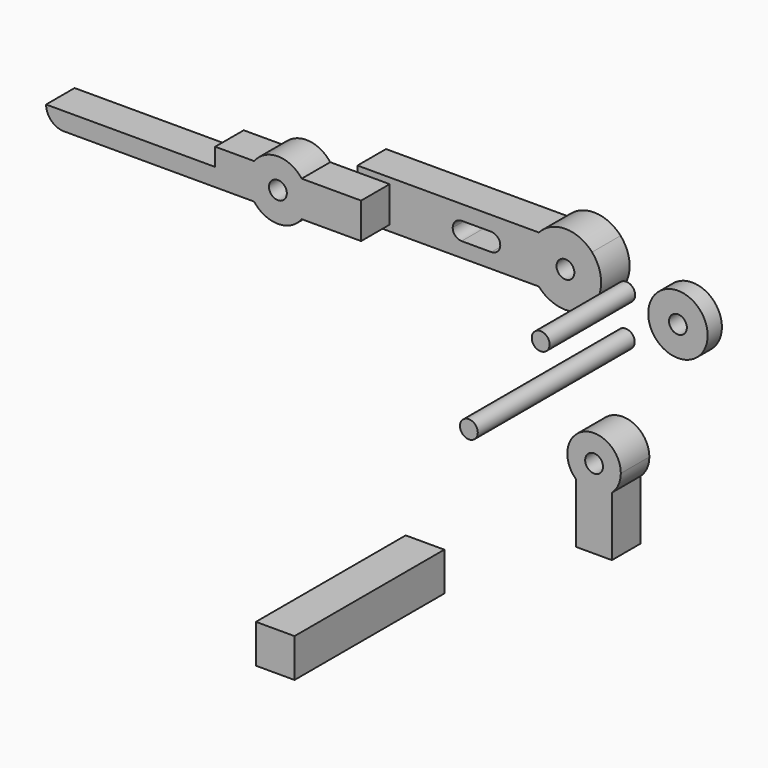
from build123d import *

# Parameters (mm, degrees)
F0_R      = 1.5
F1_DEPTH  = 6
F2_R      = 1.5
F2_W      = 5.4118521512
F2_H      = 6
F3_DEPTH  = 6
F4_R      = 5
F4_R_2    = 1.5
F5_DEPTH  = 3
F6_R      = 1.5
F7_DEPTH  = 18
F8_R      = 1.5
F9_DEPTH  = 33
F10_R     = 1.5
F10_W     = 6
F10_H     = 6
F11_DEPTH = 6
F12_DEPTH = 6
F13_W     = 6.5
F13_H     = 6.5
F14_DEPTH = 31.5


# Not quite as in the source:
# - ends of sketch curves that miss each other by under 0.0002 mm in the source are joined


with BuildPart() as f1:
    # F0 (on Front) → F1 (new body)
    with BuildSketch(Plane.XZ):
        with BuildLine():
            ThreePointArc((3.9999999804, -3.0000000261), (4.7434164851, -1.5811388455), (5, 0))
            ThreePointArc((5, 0), (4.7434164917, 1.5811388258), (4.0000000055, 2.9999999927))
            Line((3.9999999804, 2.9999999739), (3.9999999804, -3.0000000261))
        make_face()
        with BuildLine():
            ThreePointArc((4.0000000055, 2.9999999927), (4.7434164917, 1.5811388258), (5, 0))
            ThreePointArc((5, 0), (4.7434164851, -1.5811388455), (3.9999999804, -3.0000000261))
            Line((3.9999999804, -3.0000000261), (13.9999999804, -3.0000000261))
            Line((13.9999999804, -3.0000000261), (13.9999999804, 2.9999999739))
            Line((13.9999999804, 2.9999999739), (3.9999999804, 2.9999999739))
        make_face()
        with BuildLine():
            Line((3.9999999804, -3.0000000261), (3.9999999804, 2.9999999739))
            ThreePointArc((4.0000000055, 2.9999999927), (2.09e-08, 5), (-3.9999999804, 3.0000000261))
            Line((-3.9999999804, 3.0000000261), (-3.9999999804, -3.0000000261))
            ThreePointArc((-3.9999999804, -3.0000000261), (0, -5), (3.9999999804, -3.0000000261))
        make_face()
        Circle(F0_R, mode=Mode.SUBTRACT)
        with BuildLine():
            Line((-3.9999999804, -3.0000000261), (-3.9999999804, 3.0000000261))
            ThreePointArc((-3.9999999804, 3.0000000261), (-5, 0), (-3.9999999804, -3.0000000261))
        make_face()
        with BuildLine():
            ThreePointArc((-3.9999999804, -3.0000000261), (-5, 0), (-3.9999999804, 3.0000000261))
            Line((-3.9999999804, 3.0000000261), (-10.545078665, 3.0000000261))
            Line((-10.545078665, 3.0000000261), (-10.545078665, 0))
            Line((-10.545078665, 0), (-38.9999999804, 0))
            ThreePointArc((-38.9999999804, -2.61e-08), (-38.121320324, -2.1213203696), (-35.9999999804, -3.0000000261))
            Line((-35.9999999804, -3.0000000261), (-3.9999999804, -3.0000000261))
        make_face()
    extrude(amount=F1_DEPTH)

    # F2 (on face) → F3 (join)
    with BuildSketch(Plane(origin=(0, 0, 0), x_dir=(-1, 0, 0), z_dir=(0, 1, 0))):
        with BuildLine():
            ThreePointArc((-39.1041604406, 3.9999999739), (-43.5762964189, 6), (-48.0484323972, 3.9999999739))
            Line((-48.0484323972, 3.9999999739), (-39.1041604406, 3.9999999739))
        make_face()
        with BuildLine():
            Line((-39.1041606338, -4.00000019), (-48.048432204, -4.00000019))
            ThreePointArc((-48.048432204, -4.00000019), (-43.5762964189, -6), (-39.1041606338, -4.00000019))
        make_face()
        with BuildLine():
            Line((-39.1041604406, 3.9999999739), (-48.0484323972, 3.9999999739))
            ThreePointArc((-48.0484323972, 3.9999999739), (-49.5762964189, -1.449e-07), (-48.048432204, -4.00000019))
            Line((-48.048432204, -4.00000019), (-39.1041606338, -4.00000019))
            ThreePointArc((-39.1041606338, -4.00000019), (-37.9712623106, -2.1409326577), (-37.5762964189, 0))
            ThreePointArc((-37.5762964189, 0), (-37.9712622589, 2.1409325223), (-39.1041604406, 3.9999999739))
        make_face()
        with Locations((-43.5762964189, 0)):
            Circle(F2_R, mode=Mode.SUBTRACT)
        with Locations((-11.2940739049, -2.61e-08)):
            Rectangle(F2_W, F2_H)
        with BuildLine():
            Line((-8.5881474018, 3.9999999739), (-39.1041604406, 3.9999999739))
            ThreePointArc((-39.1041604406, 3.9999999739), (-37.9712622589, 2.1409325223), (-37.5762964189, 0))
            ThreePointArc((-37.5762964189, 0), (-37.9712623106, -2.1409326577), (-39.1041606338, -4.00000019))
            Line((-39.1041606338, -4.00000019), (-14.5881475508, -4.00000019))
            Line((-14.5881475508, -4.00000019), (-8.5881474018, -4.00000019))
            Line((-8.5881474018, -4.00000019), (-8.5881478293, -3.0000000261))
            Line((-8.5881478293, -3.0000000261), (-13.9999999804, -3.0000000261))
            Line((-13.9999999804, -3.0000000261), (-13.9999999804, 2.9999999739))
            Line((-13.9999999804, 2.9999999739), (-8.5881478293, 2.9999999739))
            Line((-8.5881478293, 2.9999999739), (-8.5881474018, 3.9999999739))
        make_face()
        with BuildLine():
            ThreePointArc((-24.6078900066, 1.33e-08), (-25.048135537, -1.061565088), (-26.1104506254, -1.4999978011))
            Line((-26.1104506254, -1.4999978011), (-31.1104506254, -1.4999978011))
            ThreePointArc((-31.1104506254, -1.4999978011), (-32.6104506254, 0), (-31.1104506254, 1.5))
            Line((-31.1104506254, 1.5), (-31.1104506254, 1.5137138676))
            Line((-31.1104506254, 1.5137138676), (-26.1104506254, 1.5137138676))
            Line((-26.1104506254, 1.5137138676), (-26.1104506254, 1.4999978277))
            ThreePointArc((-26.1104506254, 1.4999978277), (-25.048135537, 1.0615651145), (-24.6078900066, 1.33e-08))
        make_face(mode=Mode.SUBTRACT)
    extrude(amount=F3_DEPTH)


with BuildPart() as f5:
    # F4 (on Front) → F5 (new body)
    with BuildSketch(Plane.XZ):
        with Locations((64.899995923, 0)):
            Circle(F4_R)
        with Locations((64.899995923, 0)):
            Circle(F4_R_2, mode=Mode.SUBTRACT)
    extrude(amount=F5_DEPTH)


with BuildPart() as f7:
    # F6 (on Front) → F7 (new body)
    with BuildSketch(Plane.XZ):
        with Locations((53.8045093417, 0)):
            Circle(F6_R)
    extrude(amount=F7_DEPTH)


with BuildPart() as f9:
    # F8 (on Front) → F9 (new body)
    with BuildSketch(Plane.XZ):
        with Locations((53.7274181843, -6.9740889594)):
            Circle(F8_R)
    extrude(amount=F9_DEPTH)


with BuildPart() as f11:
    # F10 (on Front) → F11 (new body)
    with BuildSketch(Plane.XZ):
        with BuildLine():
            ThreePointArc((56.1898760498, -26.5361675613), (57.2977955124, -25.0191827928), (57.6898764372, -23.1820652485))
            ThreePointArc((57.6898764372, -23.1820652485), (51.3527593674, -19.0741459611), (50.1898760498, -26.5361668682))
            Line((50.1898760498, -26.5361668682), (50.1898760498, -26.5308583975))
            Line((50.1898760498, -26.5308583975), (56.1898760498, -26.5308583975))
            Line((56.1898760498, -26.5308583975), (56.1898760498, -26.5361675613))
        make_face()
        with Locations((53.1898764372, -23.1820652485)):
            Circle(F10_R, mode=Mode.SUBTRACT)
        with BuildLine():
            Line((50.1898760498, -26.5308583975), (50.1898760498, -26.5361668682))
            ThreePointArc((50.1898760498, -26.5361668682), (53.1898759174, -27.6820652485), (56.1898760498, -26.5361675613))
            Line((56.1898760498, -26.5361675613), (56.1898760498, -26.5308583975))
            Line((56.1898760498, -26.5308583975), (50.1898760498, -26.5308583975))
        make_face()
        with BuildLine():
            ThreePointArc((56.1898760498, -26.5361675613), (53.1898759174, -27.6820652485), (50.1898760498, -26.5361668682))
            Line((50.1898760498, -26.5361668682), (50.1898760498, -30.5308583975))
            Line((50.1898760498, -30.5308583975), (56.1898760498, -30.5308583975))
            Line((56.1898760498, -30.5308583975), (56.1898760498, -26.5361675613))
        make_face()
        with Locations((53.1898760498, -33.5308583975)):
            Rectangle(F10_W, F10_H)
    extrude(amount=F11_DEPTH)

    # F10 (on Front) → F12 (join)
    with BuildSketch(Plane.XZ):
        with BuildLine():
            ThreePointArc((56.1898760498, -26.5361675613), (57.2977955124, -25.0191827928), (57.6898764372, -23.1820652485))
            ThreePointArc((57.6898764372, -23.1820652485), (51.3527593674, -19.0741459611), (50.1898760498, -26.5361668682))
            Line((50.1898760498, -26.5361668682), (50.1898760498, -26.5308583975))
            Line((50.1898760498, -26.5308583975), (56.1898760498, -26.5308583975))
            Line((56.1898760498, -26.5308583975), (56.1898760498, -26.5361675613))
        make_face()
        with Locations((53.1898764372, -23.1820652485)):
            Circle(F10_R, mode=Mode.SUBTRACT)
        with BuildLine():
            Line((50.1898760498, -26.5308583975), (50.1898760498, -26.5361668682))
            ThreePointArc((50.1898760498, -26.5361668682), (53.1898759174, -27.6820652485), (56.1898760498, -26.5361675613))
            Line((56.1898760498, -26.5361675613), (56.1898760498, -26.5308583975))
            Line((56.1898760498, -26.5308583975), (50.1898760498, -26.5308583975))
        make_face()
        with BuildLine():
            ThreePointArc((56.1898760498, -26.5361675613), (53.1898759174, -27.6820652485), (50.1898760498, -26.5361668682))
            Line((50.1898760498, -26.5361668682), (50.1898760498, -30.5308583975))
            Line((50.1898760498, -30.5308583975), (56.1898760498, -30.5308583975))
            Line((56.1898760498, -30.5308583975), (56.1898760498, -26.5361675613))
        make_face()
        with Locations((53.1898760498, -33.5308583975)):
            Rectangle(F10_W, F10_H)
    extrude(amount=F12_DEPTH)


with BuildPart() as f14:
    # F13 (on Front) → F14 (new body)
    with BuildSketch(Plane.XZ):
        with Locations((19.9485578835, -51.390840739)):
            Rectangle(F13_W, F13_H)
    extrude(amount=F14_DEPTH)


solid = Compound([f1.part, f5.part, f7.part, f9.part, f11.part, f14.part])
